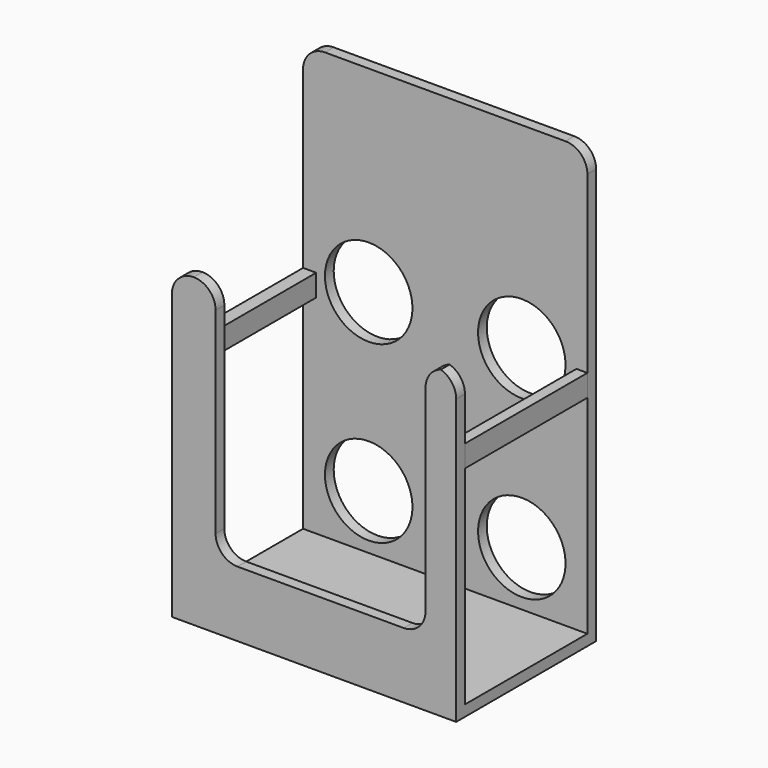
from build123d import *

# Parameters (mm, degrees)
F1_DEPTH     = 65
F2_W         = 48
F2_H         = 55
F3_DEPTH     = 10
F4_R         = 2.25
F5_DEPTH     = 5
F6_R         = 3.9
F6_R_2       = 2.25
F7_DEPTH     = 4
F8_R         = 10
F9_DEPTH     = 4
F10_W        = 35
F10_H        = 5
F11_DEPTH    = 2.5
F12_W        = 35
F12_H        = 5
F13_DEPTH    = 3
F14_T1_DEPTH = 2.5
F14_T3_DEPTH = 27.5
F14_T5_DEPTH = 27.5


# Not quite as in the source:
# - a fillet or chamfer that OpenCascade refuses, or shapes differently, is made with other operations: its cross-section is extruded or revolved along the edge and cut away or added


with BuildPart() as f1:
    # F0 (on Right) → F1 (new body)
    with BuildSketch(Plane.YZ):
        Polygon((0, -34.9315267816), (0, 65.0684732184), (-2.5, 65.0684732184), (-2.5, -32.4315267816), (-37.5, -32.4315267816), (-37.5, 35.0684732184), (-40, 35.0684732184), (-40, -34.9315267816), align=None)
    extrude(amount=F1_DEPTH)

    # F2 (on face) → F3 (cut)
    with BuildSketch(Plane.XZ.offset(40)):
        with Locations((34, 7.5684732184)):
            Rectangle(F2_W, F2_H)
    extrude(amount=-F3_DEPTH, mode=Mode.SUBTRACT)

    # F4 (on face) → F5 (join)
    with BuildSketch(Plane(origin=(0, 0, 0), x_dir=(-1, 0, 0), z_dir=(0, 1, 0))):
        with Locations((-32.5, 40.0684732184)):
            Circle(F4_R)
    extrude(amount=F5_DEPTH)

    # F6 (on face) → F7 (join)
    with BuildSketch(Plane(origin=(0, 5, 0), x_dir=(-1, 0, 0), z_dir=(0, 1, 0))):
        with Locations((-32.5, 40.0684732184)):
            Circle(F6_R)
        with Locations((-32.5, 40.0684732184)):
            Circle(F6_R_2, mode=Mode.SUBTRACT)
        with Locations((-32.5, 40.0684732184)):
            Circle(F6_R_2)
    extrude(amount=F7_DEPTH)

    # F8 (on face) → F9 (cut)
    with BuildSketch(Plane(origin=(0, 0, 0), x_dir=(-1, 0, 0), z_dir=(0, 1, 0))):
        with Locations((-50, 20.0684732184)):
            Circle(F8_R)
        with Locations((-15, 20.0684732184)):
            Circle(F8_R)
        with Locations((-15, -19.9315267816)):
            Circle(F8_R)
        with Locations((-50, -19.9315267816)):
            Circle(F8_R)
    extrude(amount=-F9_DEPTH, mode=Mode.SUBTRACT)

    # F14: fillet of radius 5 on 8 edges, made by hand

    # F14_s2 → F14_t1 (join)
    with BuildSketch(Plane.XZ.offset(37.5)):
        with BuildLine():
            ThreePointArc((15, -19.9315267816), (11.4644660941, -18.4670606876), (10, -14.9315267816))
            Line((10, -14.9315267816), (10, -19.9315267816))
            Line((10, -19.9315267816), (15, -19.9315267816))
        make_face()
        with BuildLine():
            ThreePointArc((58, -14.9315267816), (56.5355339059, -18.4670606876), (53, -19.9315267816))
            Line((53, -19.9315267816), (58, -19.9315267816))
            Line((58, -19.9315267816), (58, -14.9315267816))
        make_face()
    extrude(amount=F14_T1_DEPTH)

    # F14_s4 → F14_t3 (cut)
    with BuildSketch(Plane.XZ.offset(25)):
        with BuildLine():
            ThreePointArc((0, 30.0684732184), (1.4644660941, 33.6040071243), (5, 35.0684732184))
            Line((5, 35.0684732184), (0, 35.0684732184))
            Line((0, 35.0684732184), (0, 30.0684732184))
        make_face()
        with BuildLine():
            ThreePointArc((5, 35.0684732184), (8.5355339059, 33.6040071243), (10, 30.0684732184))
            Line((10, 30.0684732184), (10, 35.0684732184))
            Line((10, 35.0684732184), (5, 35.0684732184))
        make_face()
        with BuildLine():
            ThreePointArc((63, 35.0684732184), (59.4644660941, 33.6040071243), (58, 30.0684732184))
            Line((58, 30.0684732184), (58, 35.0684732184))
            Line((58, 35.0684732184), (63, 35.0684732184))
        make_face()
        with BuildLine():
            ThreePointArc((65, 30.0684732184), (63.5355339059, 33.6040071243), (60, 35.0684732184))
            Line((60, 35.0684732184), (65, 35.0684732184))
            Line((65, 35.0684732184), (65, 30.0684732184))
        make_face()
    extrude(amount=F14_T3_DEPTH, mode=Mode.SUBTRACT)

    # F14_s6 → F14_t5 (cut)
    with BuildSketch(Plane.XZ.offset(-12.5)):
        with BuildLine():
            ThreePointArc((65, 60.0684732184), (63.5355339059, 63.6040071243), (60, 65.0684732184))
            Line((60, 65.0684732184), (65, 65.0684732184))
            Line((65, 65.0684732184), (65, 60.0684732184))
        make_face()
        with BuildLine():
            ThreePointArc((0, 60.0684732184), (1.4644660941, 63.6040071243), (5, 65.0684732184))
            Line((5, 65.0684732184), (0, 65.0684732184))
            Line((0, 65.0684732184), (0, 60.0684732184))
        make_face()
    extrude(amount=F14_T5_DEPTH, mode=Mode.SUBTRACT)


with BuildPart() as f11:
    # F10 (on face) → F11 (new body)
    with BuildSketch(Plane.YZ.offset(65)):
        with Locations((-20, 17.5684732184)):
            Rectangle(F10_W, F10_H)
    extrude(amount=-F11_DEPTH)


with BuildPart() as f13:
    # F12 (on face) → F13 (new body)
    with BuildSketch(Plane(origin=(0, 0, 0), x_dir=(0, -1, 0), z_dir=(-1, 0, 0))):
        with Locations((20, 17.5684732184)):
            Rectangle(F12_W, F12_H)
    extrude(amount=-F13_DEPTH)


solid = Compound([f1.part, f11.part, f13.part])
